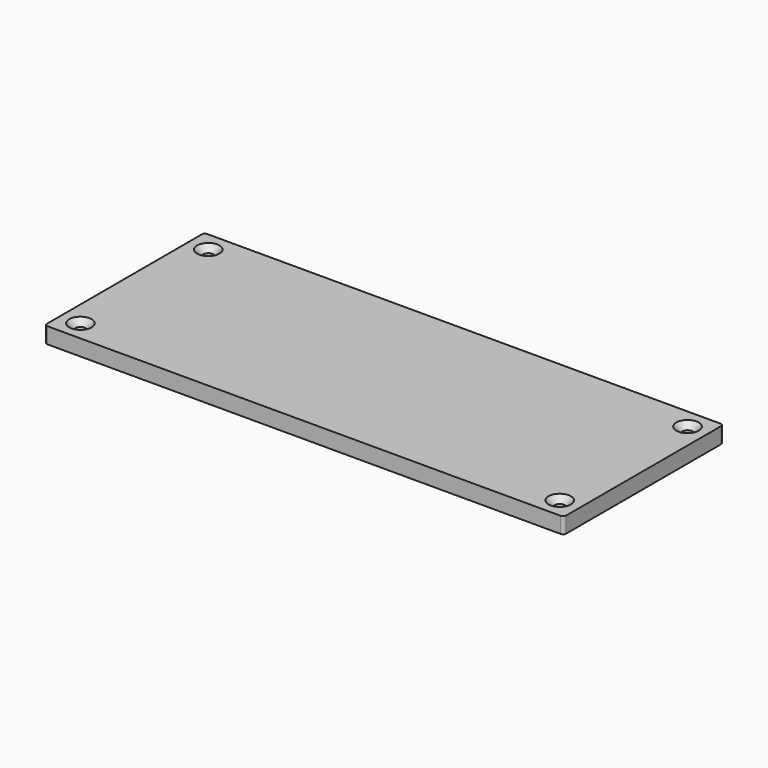
from build123d import *

# Parameters (mm, degrees)
F0_W           = 260
F0_H           = 100
F1_DEPTH       = 8
F2_D           = 5.25
F2_CSINK_D     = 11.2
F2_CSINK_ANGLE = 90
F3_R           = 1.5


# Not quite as in the source:
# - a feature names something its author has since deleted; it is built from what else it names


with BuildPart() as f1:
    # F0 (on Top) → F1 (new body)
    with BuildSketch(Plane.XY):
        with Locations((-130, 50)):
            Rectangle(F0_W, F0_H)
    extrude(amount=-F1_DEPTH)

    # F2 (through all)
    with Locations(Plane.XY):
        with Locations((-250, 10), (-10, 10), (-10, 90), (-250, 90)):
            CounterSinkHole(F2_D / 2, F2_CSINK_D / 2, counter_sink_angle=F2_CSINK_ANGLE)

    # F3
    f3_edges = [f1.edges().sort_by_distance(p)[0] for p in [
        (0, 0, -4),
        (0, 100, -4),
        (-260, 0, -4),
        (-260, 100, -4),
    ]]
    fillet(f3_edges, radius=F3_R)


solid = f1.part
